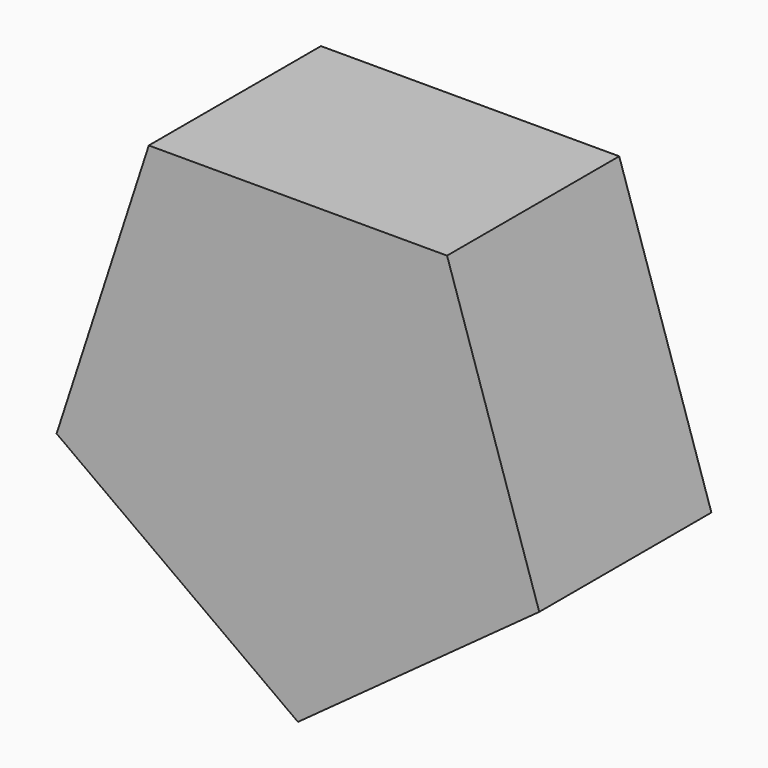
from build123d import *

# Parameters (mm, degrees)
F1_DEPTH = 22


# Not quite as in the source:
# - a feature of the source that left no trace in its solid (it failed there, or was rolled back) is left out


with BuildPart() as f1:
    # F0 (on Front) → F1 (new body)
    with BuildSketch(Plane.XZ):
        Polygon((15.2475531042, 20.986456424), (-15.2475531042, 20.986456424), (-24.6710591678, -8.0161130505), (0, -25.9406867469), (24.6710591678, -8.0161130505), align=None)
    extrude(amount=F1_DEPTH)


solid = f1.part
